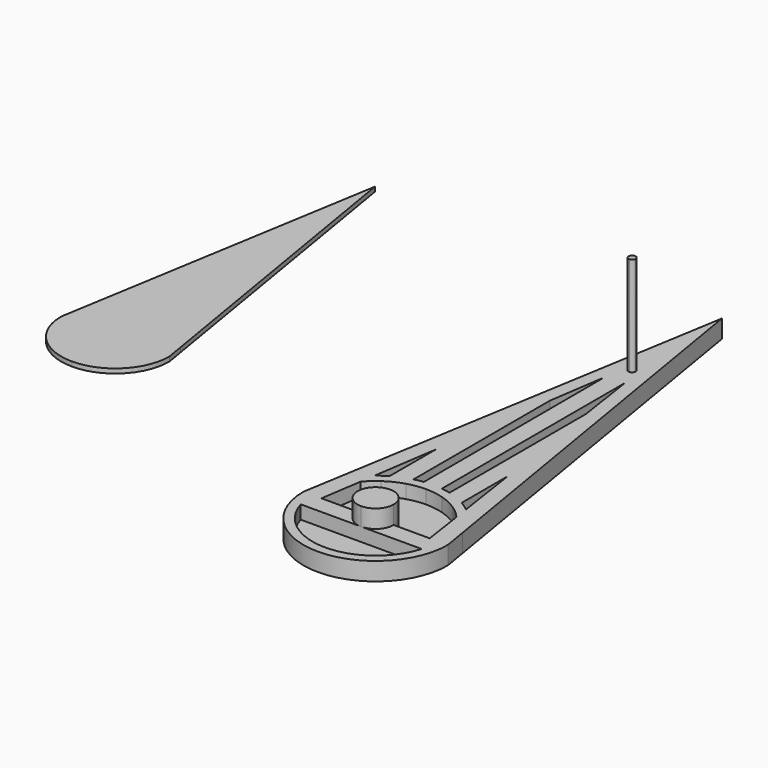
from build123d import *

# Parameters (mm, degrees)
F1_DEPTH = 3.175
F2_DEPTH = 12.7
F3_DEPTH = 3.175
F5_DEPTH = 12.7
F6_DEPTH = 82.55


with BuildPart() as f1:
    # F0 (on Top) → F1 (new body)
    with BuildSketch(Plane.XY):
        with BuildLine():
            Line((0, 0), (6.35, 0))
            ThreePointArc((6.35, 0), (7.9669082367, 11.879762203), (12.7, 22.8952505992))
            Line((12.7, 22.8952505992), (12.7, 33.6010416505))
            ThreePointArc((12.7, 33.6010416505), (6.8801890096, 25.528223647), (2.7459459459, 16.4756756757))
            Line((2.7459459459, 16.4756756757), (0, 0))
        make_face()
    extrude(amount=F1_DEPTH)



with BuildPart() as f1b:
    # F0 (on Top) → F1, piece 2 (new body)
    with BuildSketch(Plane.XY):
        with BuildLine():
            Line((95.25, 0), (101.6, 0))
            Line((101.6, 0), (98.8540540541, 16.4756756757))
            ThreePointArc((98.8540540541, 16.4756756757), (94.7198109904, 25.528223647), (88.9, 33.6010416505))
            Line((88.9, 33.6010416505), (88.9, 22.8952505992))
            ThreePointArc((88.9, 22.8952505992), (93.6330917633, 11.879762203), (95.25, 0))
        make_face()
    extrude(amount=F1_DEPTH)


with BuildPart() as f1c:
    # F0 (on Top) → F1, piece 3 (new body)
    with BuildSketch(Plane.XY):
        with BuildLine():
            Line((-243.6951210144, 106.2864051561), (-245.7545804739, 93.9296483994))
            Line((-245.7545804739, 93.9296483994), (-207.6545804739, 93.9296483994))
            Line((-207.6545804739, 93.9296483994), (-207.6545804739, 132.0296483994))
            ThreePointArc((-207.6545804739, 132.0296483994), (-229.7997556546, 124.9328936523), (-243.6951210144, 106.2864051561))
        make_face()
        with BuildLine():
            Line((-207.6545804739, 93.9296483994), (-245.7545804739, 93.9296483994))
            ThreePointArc((-245.7545804739, 93.9296483994), (-234.5953488371, 66.9888800361), (-207.6545804739, 55.8296483994))
            Line((-207.6545804739, 55.8296483994), (-207.6545804739, 93.9296483994))
        make_face()
        with BuildLine():
            Line((-207.6545804739, 93.9296483994), (-207.6545804739, 55.8296483994))
            ThreePointArc((-207.6545804739, 55.8296483994), (-180.7138121107, 66.9888800361), (-169.5545804739, 93.9296483994))
            Line((-169.5545804739, 93.9296483994), (-207.6545804739, 93.9296483994))
        make_face()
        with BuildLine():
            Line((-207.6545804739, 322.5296483994), (-243.6951210144, 106.2864051561))
            ThreePointArc((-243.6951210144, 106.2864051561), (-229.7997556546, 124.9328936523), (-207.6545804739, 132.0296483994))
            Line((-207.6545804739, 132.0296483994), (-207.6545804739, 322.5296483994))
        make_face()
        with BuildLine():
            Line((-207.6545804739, 132.0296483994), (-207.6545804739, 93.9296483994))
            Line((-207.6545804739, 93.9296483994), (-169.5545804739, 93.9296483994))
            Line((-169.5545804739, 93.9296483994), (-171.6140399334, 106.2864051561))
            ThreePointArc((-171.6140399334, 106.2864051561), (-185.5094052932, 124.9328936523), (-207.6545804739, 132.0296483994))
        make_face()
        with BuildLine():
            Line((-171.6140399334, 106.2864051561), (-207.6545804739, 322.5296483994))
            Line((-207.6545804739, 322.5296483994), (-207.6545804739, 132.0296483994))
            ThreePointArc((-207.6545804739, 132.0296483994), (-185.5094052932, 124.9328936523), (-171.6140399334, 106.2864051561))
        make_face()
    extrude(amount=F1_DEPTH)


with BuildPart() as f1_1:
    add(f1.part)

    add(f1b.part)  # F2 merges F1b
    # F0 (on Top) → F2 (join)
    with BuildSketch(Plane.XY):
        with BuildLine():
            Line((25.4, 0), (12.7, 0))
            Line((12.7, 0), (6.35, 0))
            ThreePointArc((6.35, 0), (6.8156654508, -6.4172279265), (8.2029050286, -12.7))
            Line((8.2029050286, -12.7), (50.8, -12.7))
            ThreePointArc((50.8, -12.7), (41.8197438789, -8.9802561211), (38.1, 0))
            Line((38.1, 0), (25.4, 0))
        make_face()
        with BuildLine():
            Line((6.35, 0), (12.7, 0))
            Line((12.7, 0), (12.7, 22.8952505992))
            ThreePointArc((12.7, 22.8952505992), (7.9669082367, 11.879762203), (6.35, 0))
        make_face()
        with BuildLine():
            Line((12.7, 22.8952505992), (12.7, 0))
            Line((12.7, 0), (17.0366272789, 28.9108485261))
            ThreePointArc((17.0366272789, 28.9108485261), (14.7426437559, 25.993644621), (12.7, 22.8952505992))
        make_face()
        with BuildLine():
            ThreePointArc((8.2029050286, -12.7), (6.8156654508, -6.4172279265), (6.35, 0))
            Line((6.35, 0), (0, 0))
            ThreePointArc((0, 0), (50.8, -50.8), (101.6, 0))
            Line((101.6, 0), (95.25, 0))
            ThreePointArc((95.25, 0), (94.7843345492, -6.4172279265), (93.3970949714, -12.7))
            ThreePointArc((93.3970949714, -12.7), (50.8, -44.45), (8.2029050286, -12.7))
        make_face()
        with BuildLine():
            Line((0, 0), (6.35, 0))
            ThreePointArc((6.35, 0), (7.9669082367, 11.879762203), (12.7, 22.8952505992))
            Line((12.7, 22.8952505992), (12.7, 33.6010416505))
            ThreePointArc((12.7, 33.6010416505), (6.8801890096, 25.528223647), (2.7459459459, 16.4756756757))
            Line((2.7459459459, 16.4756756757), (0, 0))
        make_face()
        with BuildLine():
            Line((12.7, 33.6010416505), (12.7, 22.8952505992))
            ThreePointArc((12.7, 22.8952505992), (14.7426437559, 25.993644621), (17.0366272789, 28.9108485261))
            Line((17.0366272789, 28.9108485261), (18.5927975033, 39.2853166888))
            ThreePointArc((18.5927975033, 39.2853166888), (15.5316937406, 36.5620920298), (12.7, 33.6010416505))
        make_face()
        with BuildLine():
            Line((18.5927975033, 39.2853166888), (17.0366272789, 28.9108485261))
            ThreePointArc((17.0366272789, 28.9108485261), (20.9773322723, 32.9607492269), (25.4, 36.4779728055))
            Line((25.4, 36.4779728055), (25.4, 43.9940905122))
            ThreePointArc((25.4, 43.9940905122), (21.9003359431, 41.7785760575), (18.5927975033, 39.2853166888))
        make_face()
        with BuildLine():
            ThreePointArc((50.8, 12.7), (41.8197438789, 8.9802561211), (38.1, 0))
            Line((38.1, 0), (50.8, 0))
            Line((50.8, 0), (50.8, 12.7))
        make_face()
        with BuildLine():
            Line((50.8, 0), (38.1, 0))
            ThreePointArc((38.1, 0), (41.8197438789, -8.9802561211), (50.8, -12.7))
            ThreePointArc((50.8, -12.7), (59.7802561211, -8.9802561211), (63.5, 0))
            Line((63.5, 0), (50.8, 0))
        make_face()
        with BuildLine():
            Line((25.4, 43.9940905122), (25.4, 36.4779728055))
            ThreePointArc((25.4, 36.4779728055), (31.5058709961, 40.0442141386), (38.1, 42.5970949714))
            Line((38.1, 42.5970949714), (38.1, 49.1868884968))
            ThreePointArc((38.1, 49.1868884968), (31.5738774651, 47.0212315053), (25.4, 43.9940905122))
        make_face()
        with BuildLine():
            Line((12.7, 76.2), (12.7, 33.6010416505))
            ThreePointArc((12.7, 33.6010416505), (15.5316937406, 36.5620920298), (18.5927975033, 39.2853166888))
            Line((18.5927975033, 39.2853166888), (25.4, 84.6666666667))
            Line((25.4, 84.6666666667), (25.4, 152.4))
            Line((25.4, 152.4), (12.7, 76.2))
        make_face()
        with BuildLine():
            ThreePointArc((2.7459459459, 16.4756756757), (6.8801890096, 25.528223647), (12.7, 33.6010416505))
            Line((12.7, 33.6010416505), (12.7, 76.2))
            Line((12.7, 76.2), (2.7459459459, 16.4756756757))
        make_face()
        with BuildLine():
            Line((50.8, 12.7), (50.8, 0))
            Line((50.8, 0), (63.5, 0))
            ThreePointArc((63.5, 0), (59.7802561211, 8.9802561211), (50.8, 12.7))
        make_face()
        with BuildLine():
            Line((38.1, 49.1868884968), (38.1, 42.5970949714))
            ThreePointArc((38.1, 42.5970949714), (44.3827720735, 43.9843345492), (50.8, 44.45))
            Line((50.8, 44.45), (50.8, 50.8))
            ThreePointArc((50.8, 50.8), (47.6187560428, 50.7002927692), (44.45, 50.4015624758))
            ThreePointArc((44.45, 50.4015624758), (41.2556570043, 49.8953456425), (38.1, 49.1868884968))
        make_face()
        with BuildLine():
            ThreePointArc((63.5, 0), (59.7802561211, -8.9802561211), (50.8, -12.7))
            Line((50.8, -12.7), (93.3970949714, -12.7))
            ThreePointArc((93.3970949714, -12.7), (94.7843345492, -6.4172279265), (95.25, 0))
            Line((95.25, 0), (88.9, 0))
            Line((88.9, 0), (76.2, 0))
            Line((76.2, 0), (63.5, 0))
        make_face()
        with BuildLine():
            Line((25.4, 84.6666666667), (25.4, 43.9940905122))
            ThreePointArc((25.4, 43.9940905122), (31.5738774651, 47.0212315053), (38.1, 49.1868884968))
            Line((38.1, 49.1868884968), (38.1, 169.3333333333))
            Line((38.1, 169.3333333333), (25.4, 84.6666666667))
        make_face()
        with BuildLine():
            Line((95.25, 0), (101.6, 0))
            Line((101.6, 0), (98.8540540541, 16.4756756757))
            ThreePointArc((98.8540540541, 16.4756756757), (94.7198109904, 25.528223647), (88.9, 33.6010416505))
            Line((88.9, 33.6010416505), (88.9, 22.8952505992))
            ThreePointArc((88.9, 22.8952505992), (93.6330917633, 11.879762203), (95.25, 0))
        make_face()
        Polygon((25.4, 152.4), (25.4, 84.6666666667), (38.1, 169.3333333333), (38.1, 228.6), align=None)
        with BuildLine():
            Line((50.8, 50.8), (50.8, 44.45))
            ThreePointArc((50.8, 44.45), (57.2172279265, 43.9843345492), (63.5, 42.5970949714))
            Line((63.5, 42.5970949714), (63.5, 49.1868884968))
            ThreePointArc((63.5, 49.1868884968), (60.3443429957, 49.8953456425), (57.15, 50.4015624758))
            ThreePointArc((57.15, 50.4015624758), (53.9812439572, 50.7002927692), (50.8, 50.8))
        make_face()
        with BuildLine():
            Line((88.9, 0), (95.25, 0))
            ThreePointArc((95.25, 0), (93.6330917633, 11.879762203), (88.9, 22.8952505992))
            Line((88.9, 22.8952505992), (88.9, 0))
        make_face()
        with BuildLine():
            ThreePointArc((88.9, 33.6010416505), (94.7198109904, 25.528223647), (98.8540540541, 16.4756756757))
            Line((98.8540540541, 16.4756756757), (88.9, 76.2))
            Line((88.9, 76.2), (88.9, 33.6010416505))
        make_face()
        with BuildLine():
            Line((38.1, 228.6), (38.1, 169.3333333333))
            Line((38.1, 169.3333333333), (44.1137143616, 209.4247624108))
            Line((44.1137143616, 209.4247624108), (45.4948143772, 218.6320958477))
            ThreePointArc((45.4948143772, 218.6320958477), (42.008355823, 227.0843623282), (47.8212586894, 234.1417245957))
            Line((47.8212586894, 234.1417245957), (50.8, 254))
            Line((50.8, 254), (50.8, 304.8))
            Line((50.8, 304.8), (38.1, 228.6))
        make_face()
        with BuildLine():
            Line((63.5, 49.1868884968), (63.5, 42.5970949714))
            ThreePointArc((63.5, 42.5970949714), (70.0941290039, 40.0442141386), (76.2, 36.4779728055))
            Line((76.2, 36.4779728055), (76.2, 43.9940905122))
            ThreePointArc((76.2, 43.9940905122), (70.0261225349, 47.0212315053), (63.5, 49.1868884968))
        make_face()
        with BuildLine():
            Line((44.1137143616, 209.4247624108), (44.45, 50.4015624758))
            ThreePointArc((44.45, 50.4015624758), (47.6187560428, 50.7002927692), (50.8, 50.8))
            Line((50.8, 50.8), (50.8, 216.8756157017))
            ThreePointArc((50.8, 216.8756157017), (48.005799891, 217.3261521079), (45.4948143772, 218.6320958477))
            Line((45.4948143772, 218.6320958477), (44.1137143616, 209.4247624108))
        make_face()
        with BuildLine():
            Line((50.8, 216.8756157017), (50.8, 50.8))
            ThreePointArc((50.8, 50.8), (53.9812439572, 50.7002927692), (57.15, 50.4015624758))
            Line((57.15, 50.4015624758), (57.15, 211.6666666667))
            Line((57.15, 211.6666666667), (56.1051856228, 218.6320958477))
            ThreePointArc((56.1051856228, 218.6320958477), (53.594200109, 217.3261521079), (50.8, 216.8756157017))
        make_face()
        with BuildLine():
            Line((84.5633727211, 28.9108485261), (88.9, 0))
            Line((88.9, 0), (88.9, 22.8952505992))
            ThreePointArc((88.9, 22.8952505992), (86.8573562441, 25.993644621), (84.5633727211, 28.9108485261))
        make_face()
        with BuildLine():
            ThreePointArc((84.5633727211, 28.9108485261), (86.8573562441, 25.993644621), (88.9, 22.8952505992))
            Line((88.9, 22.8952505992), (88.9, 33.6010416505))
            ThreePointArc((88.9, 33.6010416505), (86.0683062594, 36.5620920298), (83.0072024967, 39.2853166888))
            Line((83.0072024967, 39.2853166888), (84.5633727211, 28.9108485261))
        make_face()
        with BuildLine():
            Line((88.9, 33.6010416505), (88.9, 76.2))
            Line((88.9, 76.2), (76.2, 152.4))
            Line((76.2, 152.4), (76.2, 84.6666666667))
            Line((76.2, 84.6666666667), (83.0072024967, 39.2853166888))
            ThreePointArc((83.0072024967, 39.2853166888), (86.0683062594, 36.5620920298), (88.9, 33.6010416505))
        make_face()
        with BuildLine():
            Line((76.2, 43.9940905122), (76.2, 36.4779728055))
            ThreePointArc((76.2, 36.4779728055), (80.6226677277, 32.9607492269), (84.5633727211, 28.9108485261))
            Line((84.5633727211, 28.9108485261), (83.0072024967, 39.2853166888))
            ThreePointArc((83.0072024967, 39.2853166888), (79.6996640569, 41.7785760575), (76.2, 43.9940905122))
        make_face()
        with BuildLine():
            Line((63.5, 169.3333333333), (63.5, 49.1868884968))
            ThreePointArc((63.5, 49.1868884968), (70.0261225349, 47.0212315053), (76.2, 43.9940905122))
            Line((76.2, 43.9940905122), (76.2, 84.6666666667))
            Line((76.2, 84.6666666667), (63.5, 169.3333333333))
        make_face()
        with BuildLine():
            ThreePointArc((45.4948143772, 218.6320958477), (48.005799891, 217.3261521079), (50.8, 216.8756157017))
            Line((50.8, 216.8756157017), (50.8, 223.2656157017))
            ThreePointArc((50.8, 223.2656157017), (48.3, 225.7656157017), (50.8, 228.2656157017))
            Line((50.8, 228.2656157017), (50.8, 234.6556157017))
            ThreePointArc((50.8, 234.6556157017), (49.288627787, 234.526200958), (47.8212586894, 234.1417245957))
            Line((47.8212586894, 234.1417245957), (45.4948143772, 218.6320958477))
        make_face()
        with BuildLine():
            Line((50.8, 223.2656157017), (50.8, 216.8756157017))
            ThreePointArc((50.8, 216.8756157017), (53.594200109, 217.3261521079), (56.1051856228, 218.6320958477))
            Line((56.1051856228, 218.6320958477), (53.7787413106, 234.1417245957))
            ThreePointArc((53.7787413106, 234.1417245957), (52.311372213, 234.526200958), (50.8, 234.6556157017))
            Line((50.8, 234.6556157017), (50.8, 228.2656157017))
            ThreePointArc((50.8, 228.2656157017), (52.567766953, 227.5333826546), (53.3, 225.7656157017))
            ThreePointArc((53.3, 225.7656157017), (52.567766953, 223.9978487487), (50.8, 223.2656157017))
        make_face()
        Polygon((76.2, 84.6666666667), (76.2, 152.4), (63.5, 228.6), (63.5, 169.3333333333), align=None)
        with BuildLine():
            Line((63.5, 228.6), (50.8, 304.8))
            Line((50.8, 304.8), (50.8, 254))
            Line((50.8, 254), (53.7787413106, 234.1417245957))
            ThreePointArc((53.7787413106, 234.1417245957), (58.0633707826, 230.8915834029), (59.69, 225.7656157017))
            ThreePointArc((59.69, 225.7656157017), (58.7433997818, 221.77381161), (56.1051856228, 218.6320958477))
            Line((56.1051856228, 218.6320958477), (57.15, 211.6666666667))
            Line((57.15, 211.6666666667), (63.5, 169.3333333333))
            Line((63.5, 169.3333333333), (63.5, 228.6))
        make_face()
        with BuildLine():
            ThreePointArc((47.8212586894, 234.1417245957), (42.008355823, 227.0843623282), (45.4948143772, 218.6320958477))
            Line((45.4948143772, 218.6320958477), (47.8212586894, 234.1417245957))
        make_face()
        with BuildLine():
            Line((53.7787413106, 234.1417245957), (56.1051856228, 218.6320958477))
            ThreePointArc((56.1051856228, 218.6320958477), (58.7433997818, 221.77381161), (59.69, 225.7656157017))
            ThreePointArc((59.69, 225.7656157017), (58.0633707826, 230.8915834029), (53.7787413106, 234.1417245957))
        make_face()
        with BuildLine():
            Line((53.7787413106, 234.1417245957), (50.8, 254))
            Line((50.8, 254), (50.8, 234.6556157017))
            ThreePointArc((50.8, 234.6556157017), (52.311372213, 234.526200958), (53.7787413106, 234.1417245957))
        make_face()
        with BuildLine():
            Line((50.8, 234.6556157017), (50.8, 254))
            Line((50.8, 254), (47.8212586894, 234.1417245957))
            ThreePointArc((47.8212586894, 234.1417245957), (49.288627787, 234.526200958), (50.8, 234.6556157017))
        make_face()
    extrude(amount=F2_DEPTH)

    # F0 (on Top) → F3 (join)
    with BuildSketch(Plane.XY):
        with BuildLine():
            ThreePointArc((57.15, 50.4015624758), (60.3443429957, 49.8953456425), (63.5, 49.1868884968))
            Line((63.5, 49.1868884968), (63.5, 169.3333333333))
            Line((63.5, 169.3333333333), (57.15, 211.6666666667))
            Line((57.15, 211.6666666667), (57.15, 50.4015624758))
        make_face()
        with BuildLine():
            Line((38.1, 169.3333333333), (38.1, 49.1868884968))
            ThreePointArc((38.1, 49.1868884968), (41.2556570043, 49.8953456425), (44.45, 50.4015624758))
            Line((44.45, 50.4015624758), (44.1137143616, 209.4247624108))
            Line((44.1137143616, 209.4247624108), (38.1, 169.3333333333))
        make_face()
        with BuildLine():
            Line((25.4, 84.6666666667), (18.5927975033, 39.2853166888))
            ThreePointArc((18.5927975033, 39.2853166888), (21.9003359431, 41.7785760575), (25.4, 43.9940905122))
            Line((25.4, 43.9940905122), (25.4, 84.6666666667))
        make_face()
        with BuildLine():
            ThreePointArc((76.2, 43.9940905122), (79.6996640569, 41.7785760575), (83.0072024967, 39.2853166888))
            Line((83.0072024967, 39.2853166888), (76.2, 84.6666666667))
            Line((76.2, 84.6666666667), (76.2, 43.9940905122))
        make_face()
        with BuildLine():
            Line((25.4, 0), (12.7, 0))
            Line((12.7, 0), (6.35, 0))
            ThreePointArc((6.35, 0), (6.8156654508, -6.4172279265), (8.2029050286, -12.7))
            Line((8.2029050286, -12.7), (50.8, -12.7))
            ThreePointArc((50.8, -12.7), (41.8197438789, -8.9802561211), (38.1, 0))
            Line((38.1, 0), (25.4, 0))
        make_face()
        with BuildLine():
            Line((63.5, 42.5970949714), (63.5, 0))
            Line((63.5, 0), (76.2, 0))
            Line((76.2, 0), (76.2, 36.4779728055))
            ThreePointArc((76.2, 36.4779728055), (70.0941290039, 40.0442141386), (63.5, 42.5970949714))
        make_face()
        with BuildLine():
            Line((76.2, 36.4779728055), (76.2, 0))
            Line((76.2, 0), (88.9, 0))
            Line((88.9, 0), (84.5633727211, 28.9108485261))
            ThreePointArc((84.5633727211, 28.9108485261), (80.6226677277, 32.9607492269), (76.2, 36.4779728055))
        make_face()
        with BuildLine():
            Line((17.0366272789, 28.9108485261), (12.7, 0))
            Line((12.7, 0), (25.4, 0))
            Line((25.4, 0), (25.4, 36.4779728055))
            ThreePointArc((25.4, 36.4779728055), (20.9773322723, 32.9607492269), (17.0366272789, 28.9108485261))
        make_face()
        with BuildLine():
            Line((25.4, 36.4779728055), (25.4, 0))
            Line((25.4, 0), (38.1, 0))
            Line((38.1, 0), (38.1, 42.5970949714))
            ThreePointArc((38.1, 42.5970949714), (31.5058709961, 40.0442141386), (25.4, 36.4779728055))
        make_face()
        with BuildLine():
            Line((38.1, 42.5970949714), (38.1, 0))
            ThreePointArc((38.1, 0), (41.8197438789, 8.9802561211), (50.8, 12.7))
            Line((50.8, 12.7), (50.8, 44.45))
            ThreePointArc((50.8, 44.45), (44.3827720735, 43.9843345492), (38.1, 42.5970949714))
        make_face()
        with BuildLine():
            Line((50.8, 44.45), (50.8, 12.7))
            ThreePointArc((50.8, 12.7), (59.7802561211, 8.9802561211), (63.5, 0))
            Line((63.5, 0), (63.5, 42.5970949714))
            ThreePointArc((63.5, 42.5970949714), (57.2172279265, 43.9843345492), (50.8, 44.45))
        make_face()
        with BuildLine():
            Line((50.8, -12.7), (8.2029050286, -12.7))
            ThreePointArc((8.2029050286, -12.7), (50.8, -44.45), (93.3970949714, -12.7))
            Line((93.3970949714, -12.7), (50.8, -12.7))
        make_face()
        with BuildLine():
            Line((53.7787413106, 234.1417245957), (56.1051856228, 218.6320958477))
            ThreePointArc((56.1051856228, 218.6320958477), (58.7433997818, 221.77381161), (59.69, 225.7656157017))
            ThreePointArc((59.69, 225.7656157017), (58.0633707826, 230.8915834029), (53.7787413106, 234.1417245957))
        make_face()
        with BuildLine():
            Line((50.8, 223.2656157017), (50.8, 216.8756157017))
            ThreePointArc((50.8, 216.8756157017), (53.594200109, 217.3261521079), (56.1051856228, 218.6320958477))
            Line((56.1051856228, 218.6320958477), (53.7787413106, 234.1417245957))
            ThreePointArc((53.7787413106, 234.1417245957), (52.311372213, 234.526200958), (50.8, 234.6556157017))
            Line((50.8, 234.6556157017), (50.8, 228.2656157017))
            ThreePointArc((50.8, 228.2656157017), (52.567766953, 227.5333826546), (53.3, 225.7656157017))
            ThreePointArc((53.3, 225.7656157017), (52.567766953, 223.9978487487), (50.8, 223.2656157017))
        make_face()
        with BuildLine():
            ThreePointArc((45.4948143772, 218.6320958477), (48.005799891, 217.3261521079), (50.8, 216.8756157017))
            Line((50.8, 216.8756157017), (50.8, 223.2656157017))
            ThreePointArc((50.8, 223.2656157017), (48.3, 225.7656157017), (50.8, 228.2656157017))
            Line((50.8, 228.2656157017), (50.8, 234.6556157017))
            ThreePointArc((50.8, 234.6556157017), (49.288627787, 234.526200958), (47.8212586894, 234.1417245957))
            Line((47.8212586894, 234.1417245957), (45.4948143772, 218.6320958477))
        make_face()
        with BuildLine():
            ThreePointArc((47.8212586894, 234.1417245957), (42.008355823, 227.0843623282), (45.4948143772, 218.6320958477))
            Line((45.4948143772, 218.6320958477), (47.8212586894, 234.1417245957))
        make_face()
        with BuildLine():
            Line((53.7787413106, 234.1417245957), (50.8, 254))
            Line((50.8, 254), (50.8, 234.6556157017))
            ThreePointArc((50.8, 234.6556157017), (52.311372213, 234.526200958), (53.7787413106, 234.1417245957))
        make_face()
        with BuildLine():
            Line((50.8, 234.6556157017), (50.8, 254))
            Line((50.8, 254), (47.8212586894, 234.1417245957))
            ThreePointArc((47.8212586894, 234.1417245957), (49.288627787, 234.526200958), (50.8, 234.6556157017))
        make_face()
    extrude(amount=F3_DEPTH)

    # F4 (on face) → F5 (join)
    with BuildSketch(Plane.XY.offset(12.7)):
        with BuildLine():
            ThreePointArc((50.8, -12.7), (59.7802561211, -8.9802561211), (63.5, 0))
            ThreePointArc((63.5, 0), (50.8, 12.7), (38.1, 0))
            ThreePointArc((38.1, 0), (41.8197438789, -8.9802561211), (50.8, -12.7))
        make_face()
    extrude(amount=F5_DEPTH)

    # F0 (on Top) → F6 (join)
    with BuildSketch(Plane.XY):
        with BuildLine():
            Line((50.8, 228.2656157017), (50.8, 223.2656157017))
            ThreePointArc((50.8, 223.2656157017), (52.567766953, 223.9978487487), (53.3, 225.7656157017))
            ThreePointArc((53.3, 225.7656157017), (52.567766953, 227.5333826546), (50.8, 228.2656157017))
        make_face()
        with BuildLine():
            ThreePointArc((50.8, 228.2656157017), (48.3, 225.7656157017), (50.8, 223.2656157017))
            Line((50.8, 223.2656157017), (50.8, 228.2656157017))
        make_face()
    extrude(amount=F6_DEPTH)


solid = Compound([f1c.part, f1_1.part])
